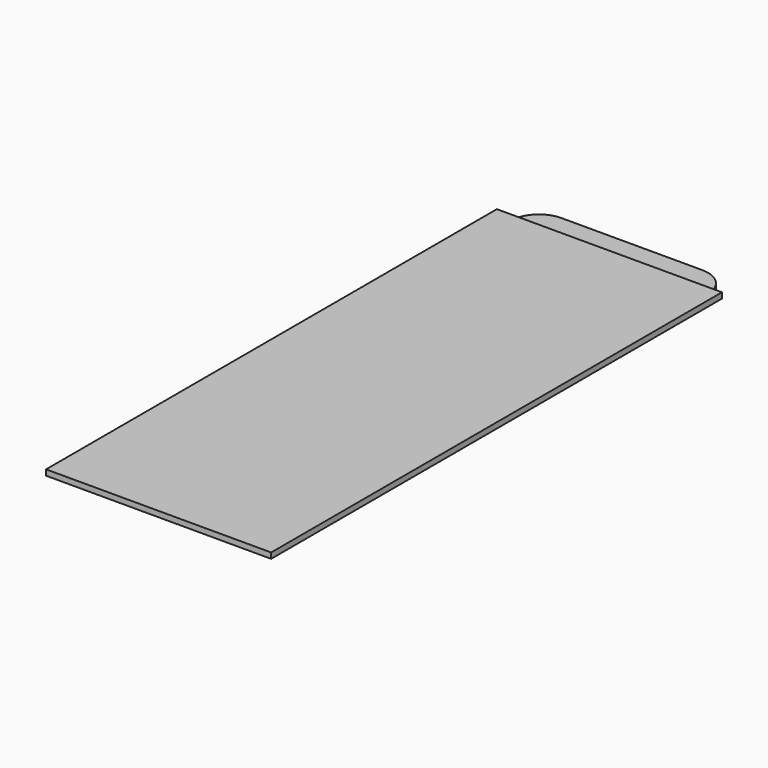
from build123d import *

# Parameters (mm, degrees)
F0_W         = 35
F0_H         = 5
F1_DEPTH     = 1
F2_DEPTH     = 1.2
F3_W         = 5
F3_H         = 85
F4_DEPTH     = 2
F5_T4_DEPTH  = 99.1421356237
F5_T9_DEPTH  = 99.1421356237
F5_T14_DEPTH = 99.1421356237
F5_T19_DEPTH = 99.1421356237
F5_T24_DEPTH = 99.1421356237
F5_T29_DEPTH = 99.1421356237
F5_T34_DEPTH = 99.1421356237
F5_T39_DEPTH = 99.1421356237
F6_R         = 5


# Not quite as in the source:
# - a fillet or chamfer that OpenCascade refuses, or shapes differently, is made with other operations: its cross-section is extruded or revolved along the edge and cut away or added


with BuildPart() as f1:
    # F0 (on Top) → F1 (new body)
    with BuildSketch(Plane.XY):
        Polygon((-19.95, -49.95), (19.95, -49.95), (19.95, 49.95), (17.5, 49.95), (17.5, 44.95), (-17.5, 44.95), (-17.5, 49.95), (-19.95, 49.95), align=None)
        with Locations((0, 47.45)):
            Rectangle(F0_W, F0_H)
    extrude(amount=F1_DEPTH)

    # F0 (on Top) → F2 (join)
    with BuildSketch(Plane.XY):
        with Locations((0, 52.45)):
            Rectangle(F0_W, F0_H)
        with Locations((0, 47.45)):
            Rectangle(F0_W, F0_H)
    extrude(amount=-F2_DEPTH)

    # F3 (on face) → F4 (join)
    with BuildSketch(Plane.XY):
        with Locations((-12.45, 2.55)):
            Rectangle(F3_W, F3_H)
        with Locations((12.45, 2.55)):
            Rectangle(F3_W, F3_H)
    extrude(amount=-F4_DEPTH)

    # F5: fillet of radius 3 on 4 edges, made by hand


with BuildPart() as f5_tool2:
    # F5_s3 → F5_t4 (new body)
    with BuildSketch(Plane.XZ.offset(-52.1210678119)):
        with BuildLine():
            ThreePointArc((-14.95, 0), (-13.8536236828, -1.4494897428), (-12.1215728753, -2))
            Line((-12.1215728753, -2), (-14.95, -2))
            Line((-14.95, -2), (-14.95, 0))
        make_face()
    extrude(amount=F5_T4_DEPTH)

    split(bisect_by=Plane.XY.offset(-1.2), keep=Keep.BOTTOM)


with BuildPart() as f1_1:
    add(f1.part)

    # F5_t1: cut F5_tool2
    add(f5_tool2.part, mode=Mode.SUBTRACT)


with BuildPart() as f5_tool7:
    # F5_s8 → F5_t9 (new body)
    with BuildSketch(Plane.XZ.offset(-52.1210678119)):
        with BuildLine():
            ThreePointArc((-14.95, 0), (-13.8536236828, -1.4494897428), (-12.1215728753, -2))
            Line((-12.1215728753, -2), (-14.95, -2))
            Line((-14.95, -2), (-14.95, 0))
        make_face()
    extrude(amount=F5_T9_DEPTH)

    split(bisect_by=Plane.XZ.offset(-44.95), keep=Keep.TOP)


with BuildPart() as f1_2:
    add(f1_1.part)

    # F5_t6: cut F5_tool7
    add(f5_tool7.part, mode=Mode.SUBTRACT)


with BuildPart() as f5_tool12:
    # F5_s13 → F5_t14 (new body)
    with BuildSketch(Plane.XZ.offset(47.0210678119)):
        with BuildLine():
            ThreePointArc((-9.95, 0), (-11.0463763172, -1.4494897428), (-12.7784271247, -2))
            Line((-12.7784271247, -2), (-9.95, -2))
            Line((-9.95, -2), (-9.95, 0))
        make_face()
    extrude(amount=-F5_T14_DEPTH)

    split(bisect_by=Plane.XZ.offset(-44.95), keep=Keep.TOP)


with BuildPart() as f1_3:
    add(f1_2.part)

    # F5_t11: cut F5_tool12
    add(f5_tool12.part, mode=Mode.SUBTRACT)


with BuildPart() as f5_tool17:
    # F5_s18 → F5_t19 (new body)
    with BuildSketch(Plane.XZ.offset(47.0210678119)):
        with BuildLine():
            ThreePointArc((-9.95, 0), (-11.0463763172, -1.4494897428), (-12.7784271247, -2))
            Line((-12.7784271247, -2), (-9.95, -2))
            Line((-9.95, -2), (-9.95, 0))
        make_face()
    extrude(amount=-F5_T19_DEPTH)

    split(bisect_by=Plane.XY.offset(-1.2), keep=Keep.BOTTOM)


with BuildPart() as f1_4:
    add(f1_3.part)

    # F5_t16: cut F5_tool17
    add(f5_tool17.part, mode=Mode.SUBTRACT)


with BuildPart() as f5_tool22:
    # F5_s23 → F5_t24 (new body)
    with BuildSketch(Plane.XZ.offset(47.0210678119)):
        with BuildLine():
            ThreePointArc((14.95, 0), (13.8536236828, -1.4494897428), (12.1215728753, -2))
            Line((12.1215728753, -2), (14.95, -2))
            Line((14.95, -2), (14.95, 0))
        make_face()
    extrude(amount=-F5_T24_DEPTH)

    split(bisect_by=Plane.XZ.offset(-44.95), keep=Keep.TOP)


with BuildPart() as f1_5:
    add(f1_4.part)

    # F5_t21: cut F5_tool22
    add(f5_tool22.part, mode=Mode.SUBTRACT)


with BuildPart() as f5_tool27:
    # F5_s28 → F5_t29 (new body)
    with BuildSketch(Plane.XZ.offset(47.0210678119)):
        with BuildLine():
            ThreePointArc((14.95, 0), (13.8536236828, -1.4494897428), (12.1215728753, -2))
            Line((12.1215728753, -2), (14.95, -2))
            Line((14.95, -2), (14.95, 0))
        make_face()
    extrude(amount=-F5_T29_DEPTH)

    split(bisect_by=Plane.XY.offset(-1.2), keep=Keep.BOTTOM)


with BuildPart() as f1_6:
    add(f1_5.part)

    # F5_t26: cut F5_tool27
    add(f5_tool27.part, mode=Mode.SUBTRACT)


with BuildPart() as f5_tool32:
    # F5_s33 → F5_t34 (new body)
    with BuildSketch(Plane.XZ.offset(-52.1210678119)):
        with BuildLine():
            ThreePointArc((9.95, 0), (11.0463763172, -1.4494897428), (12.7784271247, -2))
            Line((12.7784271247, -2), (9.95, -2))
            Line((9.95, -2), (9.95, 0))
        make_face()
    extrude(amount=F5_T34_DEPTH)

    split(bisect_by=Plane.XY.offset(-1.2), keep=Keep.BOTTOM)


with BuildPart() as f1_7:
    add(f1_6.part)

    # F5_t31: cut F5_tool32
    add(f5_tool32.part, mode=Mode.SUBTRACT)


with BuildPart() as f5_tool37:
    # F5_s38 → F5_t39 (new body)
    with BuildSketch(Plane.XZ.offset(-52.1210678119)):
        with BuildLine():
            ThreePointArc((9.95, 0), (11.0463763172, -1.4494897428), (12.7784271247, -2))
            Line((12.7784271247, -2), (9.95, -2))
            Line((9.95, -2), (9.95, 0))
        make_face()
    extrude(amount=F5_T39_DEPTH)

    split(bisect_by=Plane.XZ.offset(-44.95), keep=Keep.TOP)


with BuildPart() as f1_8:
    add(f1_7.part)

    # F5_t36: cut F5_tool37
    add(f5_tool37.part, mode=Mode.SUBTRACT)

    # F6
    f6_edges = [f1_8.edges().sort_by_distance(p)[0] for p in [
        (-17.5, 54.95, -0.6),
        (17.5, 54.95, -0.6),
    ]]
    fillet(f6_edges, radius=F6_R)


solid = f1_8.part
